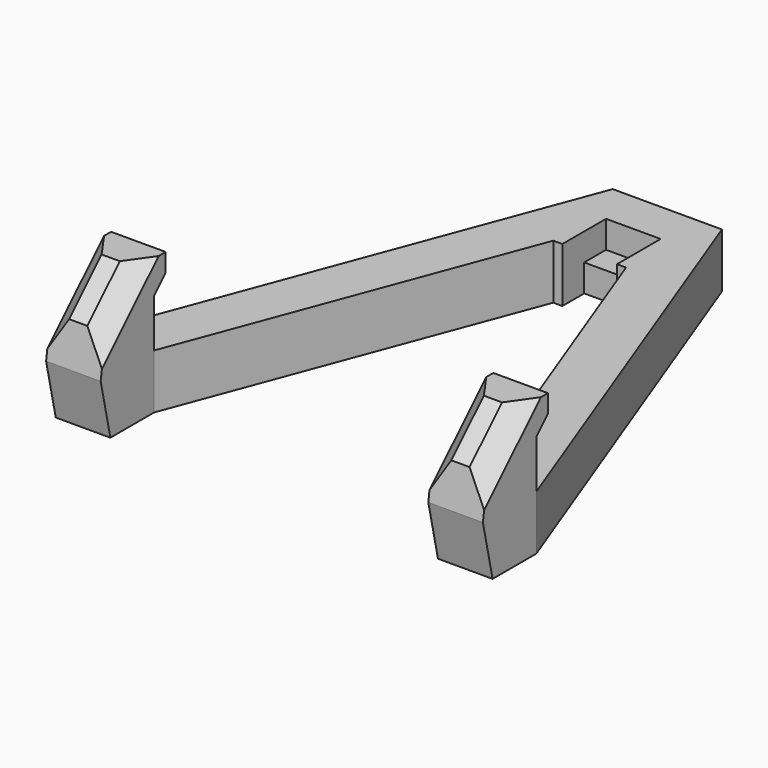
from build123d import *

# Parameters (mm, degrees)
F1_DEPTH = 9.525
F3_DEPTH = 9.525
F4_W     = 9.525
F4_H     = 9.525
F5_DEPTH = 4.7625
F6_W     = 9.525
F6_H     = 4.7625
F7_DEPTH = 4.7635
F8_SIZE  = 3.175


# Not quite as in the source:
# - a pattern or mirror of a feature is missing from the dataset's text; its kind, count and spacing are read off the source's solid


with BuildPart() as f1:
    # F0 (on Top) → F1 (new body)
    with BuildSketch(Plane.XY):
        Polygon((9.525, 0), (0, 0), (-9.525, 0), (-38.1, -76.2), (-38.1, -85.725), (-28.575, -85.725), (-28.575, -76.2), (-6.35, -16.9333333333), (0, -16.9333333333), (6.35, -16.9333333333), (28.575, -76.2), (28.575, -85.725), (38.1, -85.725), (38.1, -76.2), align=None)
    extrude(amount=F1_DEPTH)

    # F2 (on face) → F3 (join)
    with BuildSketch(Plane.YZ.offset(38.1)):
        Polygon((-85.725, 9.525), (-76.2, 9.525), (-76.2, 17.907), (-76.2, 20.447), (-73.66, 20.447), (-73.66, 23.622), (-79.6925, 23.622), (-86.7808208308, 16.5735), (-87.8366416617, 9.525), (-85.725, 0), align=None)
        Polygon((-76.2, 20.447), (-76.2, 17.907), (-73.66, 20.447), align=None)
    f3 = extrude(amount=-F3_DEPTH)

    # F3_copies: F3 across plane
    add(f3.mirror(Plane(origin=(0, 0, 0), x_dir=(0, 0, -1), z_dir=(-1, 0, 0))))

    # F4 (on face) → F5 (cut)
    with BuildSketch(Plane.XY.offset(9.525)):
        with Locations((0, -12.1708333333)):
            Rectangle(F4_W, F4_H)
    extrude(amount=-F5_DEPTH, mode=Mode.SUBTRACT)

    # F6 (on face) → F7 (cut, through all)
    with BuildSketch(Plane.XY.offset(4.7625)):
        with Locations((0, -14.5520833333)):
            Rectangle(F6_W, F6_H)
    extrude(amount=-F7_DEPTH, mode=Mode.SUBTRACT)

    # F8
    f8_edges = [f1.edges().sort_by_distance(p)[0] for p in [
        (38.1, -83.23666, 20.09775),
        (28.575, -83.23666, 20.09775),
        (-38.1, -83.23666, 20.09775),
        (-28.575, -83.23666, 20.09775),
    ]]
    chamfer(f8_edges, length=F8_SIZE)


solid = f1.part
